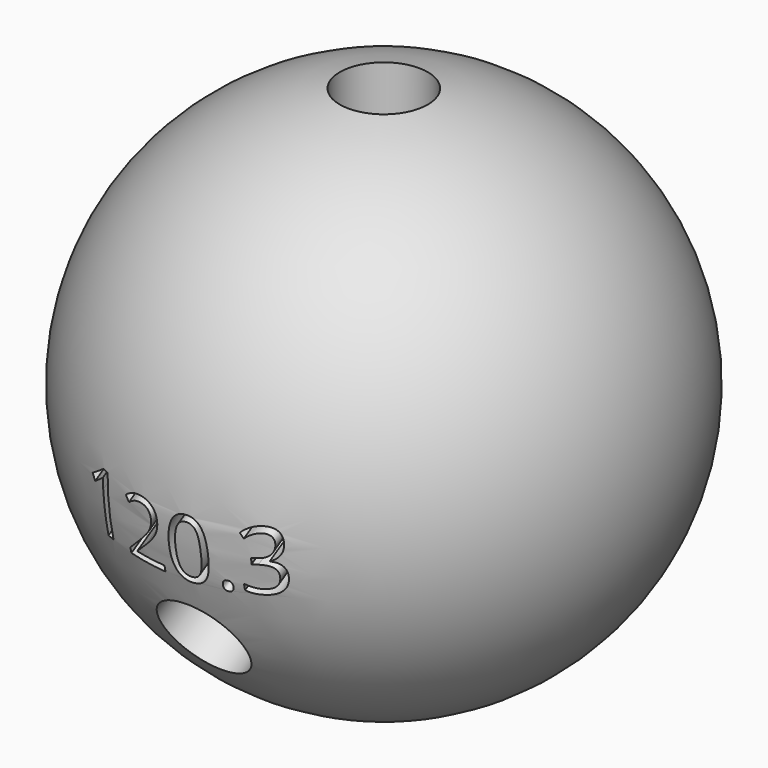
from build123d import *

# Parameters (mm, degrees)
F5_R          = 3.175
F6_DEPTH      = 76.2
F7_ANGLE      = 120.3
F8_ANGLE      = 119
F10_TEXT_SIZE = 5.7784387738
F11_DEPTH     = 6.35
F13_TEXT_SIZE = 6.645384969
F14_DEPTH     = 6.35


# Not quite as in the source:
# - Text() gives the source's letters only with a copy of the font that has no kerning and outlines rounded to 1/6400 em; it was checked with that copy


with BuildPart() as f2:
    # F0 (on Front) → F2 (revolve)
    with BuildSketch(Plane.XZ):
        with BuildLine():
            Line((0, -19.05), (0, 19.05))
            ThreePointArc((0, 19.05), (-19.05, 0), (0, -19.05))
        make_face()
    revolve(axis=Axis((0, 0, 0), (0, 0, 1)))

    # F10 (on offset) → F11 (cut)
    with BuildSketch(Plane(origin=(0, -17.5441975883, -10.2520013159), x_dir=(1, 0, 0), z_dir=(0, -0.8633955506, -0.5045276238))):
        with Locations((-7.3158596642, 5.1700836048)):
            Text('120.3', F10_TEXT_SIZE, font='Open Sans', text_align=(TextAlign.LEFT, TextAlign.BOTTOM))
    extrude(amount=-F11_DEPTH, mode=Mode.SUBTRACT)

    # F13 (on offset) → F14 (cut)
    with BuildSketch(Plane(origin=(0, 17.4721981588, -10.374232092), x_dir=(-1, 0, 0), z_dir=(0, 0.8598522716, -0.5105429179))):
        with Locations((-5.7363170721, 4.5067444444)):
            Text('119', F13_TEXT_SIZE, font='Open Sans', text_align=(TextAlign.LEFT, TextAlign.BOTTOM))
    extrude(amount=-F14_DEPTH, mode=Mode.SUBTRACT)


with BuildPart() as f6:
    # F5 (on offset) → F6 (new body)
    with BuildSketch(Plane.XY.offset(7.62)):
        Circle(F5_R)
    extrude(amount=F6_DEPTH)


with BuildPart() as f7_1:
    # F7: copy of F6
    add(f6.part.rotate(Axis((38.1614528596, 0, 0), (1, 0, 0)), F7_ANGLE))


with BuildPart() as f8_1:
    # F8: copy of F7_1
    add(f7_1.part.rotate(Axis((38.1614528596, 0, 0), (1, 0, 0)), F8_ANGLE))


with BuildPart() as f2_1:
    add(f2.part)

    # F15: cut F6, F7_1, F8_1
    add(f6.part, mode=Mode.SUBTRACT)
    add(f7_1.part, mode=Mode.SUBTRACT)
    add(f8_1.part, mode=Mode.SUBTRACT)


solid = f2_1.part
